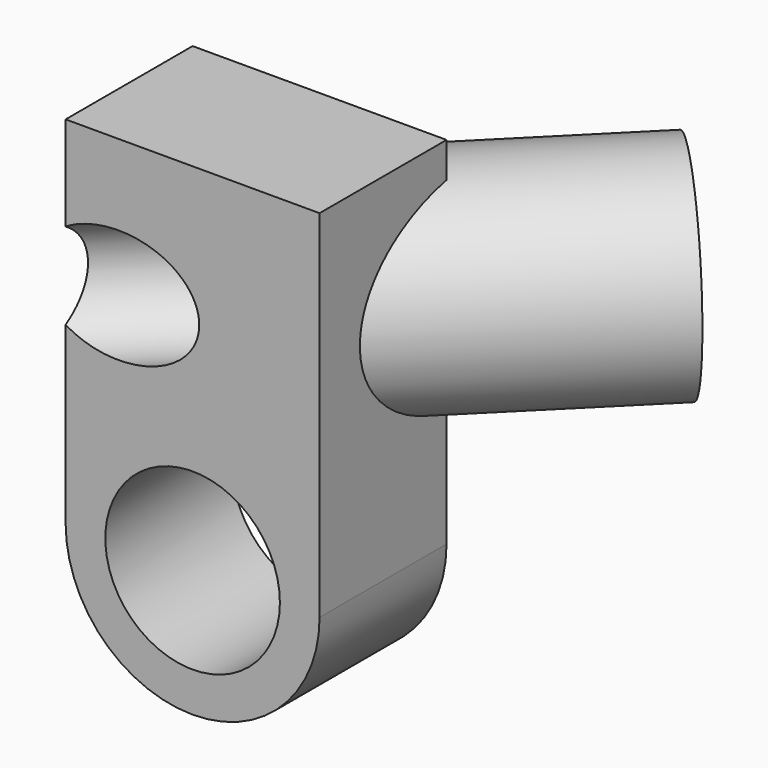
from build123d import *

# Parameters (mm, degrees)
F1_DEPTH      = 5
F4_R          = 1.8
F5_DEPTH      = 25
F4_R_2        = 3.3576804347
F6_DEPTH      = 5
F6_DEPTH_BACK = 5.36


with BuildPart() as f1:
    # F0 (on Front) → F1 (new body)
    with BuildSketch(Plane.XZ):
        with BuildLine():
            ThreePointArc((-4, 0), (0, 4), (4, 0))
            Line((4, 0), (4, 11.2083284184))
            Line((4, 11.2083284184), (-4, 11.2083284184))
            Line((-4, 11.2083284184), (-4, 0))
        make_face()
        with BuildLine():
            Line((4, 0), (2.75, 0))
            ThreePointArc((2.75, 0), (0, -2.75), (-2.75, 0))
            Line((-2.75, 0), (-4, 0))
            ThreePointArc((-4, 0), (0, -4), (4, 0))
        make_face()
        with BuildLine():
            ThreePointArc((-2.75, 0), (0, 2.75), (2.75, 0))
            Line((2.75, 0), (4, 0))
            ThreePointArc((4, 0), (0, 4), (-4, 0))
            Line((-4, 0), (-2.75, 0))
        make_face()
    extrude(amount=F1_DEPTH)

    # F4 (on face) → F5 (cut)
    with BuildSketch(Plane(origin=(2.7526911935, 2.7526911935, 0), x_dir=(-0.7071067812, 0.7071067812, 0), z_dir=(0.7071067812, 0.7071067812, 0))):
        with Locations((-1.8839619588, 6.8741668947)):
            Circle(F4_R)
    extrude(amount=-F5_DEPTH, mode=Mode.SUBTRACT)

    # F4 (on face) → F6 (join, two sides)
    with BuildSketch(Plane(origin=(2.7526911935, 2.7526911935, 0), x_dir=(-0.7071067812, 0.7071067812, 0), z_dir=(0.7071067812, 0.7071067812, 0))) as f6_sk:
        with Locations((-1.8839619588, 6.8741668947)):
            Circle(F4_R_2)
        with Locations((-1.8839619588, 6.8741668947)):
            Circle(F4_R, mode=Mode.SUBTRACT)
    extrude(amount=F6_DEPTH)
    extrude(f6_sk.sketch, amount=-F6_DEPTH_BACK)


solid = f1.part
